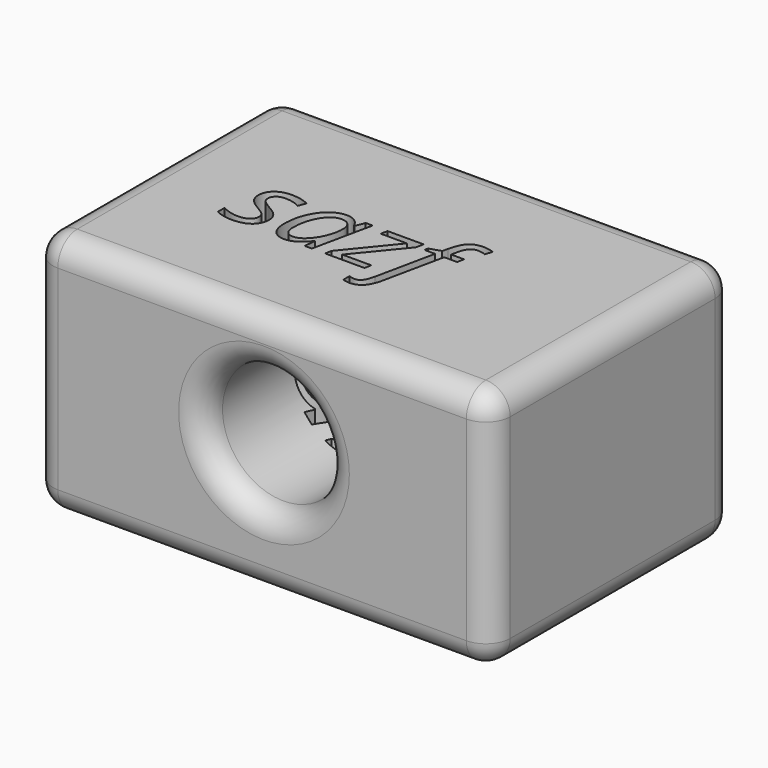
from build123d import *

# Parameters (mm, degrees)
F0_W         = 150
F0_H         = 80
F0_R         = 20
F1_DEPTH     = 50
F2_TEXT_SIZE = 36.7943572605
F3_DEPTH     = 60
F4_R         = 8


# Not quite as in the source:
# - Text() gives the source's letters only with a copy of the font that has no kerning and outlines rounded to 1/6400 em; it was checked with that copy


with BuildPart() as f1:
    # F0 (on Front) → F1 (new body, symmetric)
    with BuildSketch(Plane.XZ):
        with Locations((-0.6350819021, -3.4901006228)):
            Rectangle(F0_W, F0_H)
        Circle(F0_R, mode=Mode.SUBTRACT)
    extrude(amount=F1_DEPTH, both=True)

    # F2 (on face) → F3 (cut)
    with BuildSketch(Plane.XY.offset(36.5098993772)):
        with Locations((-45.6804446876, -12.8830652684)):
            Text('sazf', F2_TEXT_SIZE, font='Open Sans', font_style=FontStyle.ITALIC, text_align=(TextAlign.LEFT, TextAlign.BOTTOM))
    extrude(amount=-F3_DEPTH, mode=Mode.SUBTRACT)

    # F4
    f4_edges = [f1.edges().sort_by_distance(p)[0] for p in [
        (74.364918, 50, -3.490101),
        (-0.635082, 50, 36.509899),
        (-75.635082, 50, -3.490101),
        (-0.635082, 50, -43.490101),
        (-20, 50, 0),
        (74.364918, 0, 36.509899),
        (74.364918, -50, -3.490101),
        (74.364918, 0, -43.490101),
        (-0.635082, -50, 36.509899),
        (-75.635082, -50, -3.490101),
        (-0.635082, -50, -43.490101),
        (-20, -50, 0),
        (-75.635082, 0, 36.509899),
        (-75.635082, 0, -43.490101),
    ]]
    fillet(f4_edges, radius=F4_R)


solid = f1.part
